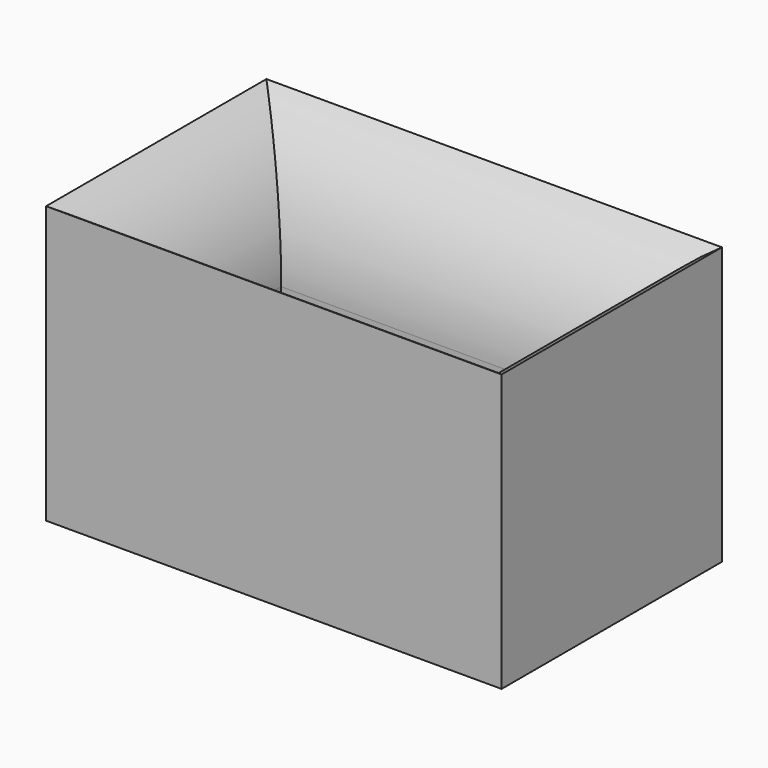
from build123d import *

# Parameters (mm, degrees)
F0_W         = 77.9829304665
F0_H         = 47.1442025155
F1_DEPTH     = 50.8
F2_T         = -12.7
F3_T1_DEPTH  = 52.5829304665
F3_T3_DEPTH  = 21.7442025155
F3_T9_DEPTH  = 116.0829304665
F3_T15_DEPTH = 85.2442025155
F3_T24_DEPTH = 116.0829304665
F3_T30_DEPTH = 85.2442025155
F3_T39_DEPTH = 116.0829304665
F3_T45_DEPTH = 85.2442025155
F3_T54_DEPTH = 85.2442025155
F3_T60_DEPTH = 116.0829304665


# Not quite as in the source:
# - a fillet or chamfer that OpenCascade refuses, or shapes differently, is made with other operations: its cross-section is extruded or revolved along the edge and cut away or added


with BuildPart() as f1:
    # F0 (on Top) → F1 (new body)
    with BuildSketch(Plane.XY):
        with Locations((25.9893098846, -0.1163231209)):
            Rectangle(F0_W, F0_H)
    extrude(amount=F1_DEPTH)

    # F2
    f2_openings = [f1.faces().sort_by_distance(p)[0] for p in [
        (25.98931, -0.116323, 50.8),
    ]]
    offset(amount=F2_T, openings=f2_openings)

    # F3: fillet of radius 25.4 on 4 edges, made by hand

    # F3_s2 → F3_t1 (cut)
    with BuildSketch(Plane.YZ.offset(-0.3021553487)):
        with BuildLine():
            ThreePointArc((36.1557781368, 50.8), (18.1952658947, 43.3605122421), (10.7557781368, 25.4))
            Line((10.7557781368, 25.4), (10.7557781368, 50.8))
            Line((10.7557781368, 50.8), (36.1557781368, 50.8))
        make_face()
        with BuildLine():
            ThreePointArc((-36.3884243786, 50.8), (-18.4279121365, 43.3605122421), (-10.9884243786, 25.4))
            Line((-10.9884243786, 25.4), (-10.9884243786, 50.8))
            Line((-10.9884243786, 50.8), (-36.3884243786, 50.8))
        make_face()
    extrude(amount=F3_T1_DEPTH, mode=Mode.SUBTRACT)

    # F3_s4 → F3_t3 (cut)
    with BuildSketch(Plane.XZ.offset(-10.7557781368)):
        with BuildLine():
            ThreePointArc((-25.7021553487, 50.8), (-7.7416431065, 43.3605122421), (-0.3021553487, 25.4))
            Line((-0.3021553487, 25.4), (-0.3021553487, 50.8))
            Line((-0.3021553487, 50.8), (-25.7021553487, 50.8))
        make_face()
        with BuildLine():
            ThreePointArc((77.6807751179, 50.8), (59.7202628757, 43.3605122421), (52.2807751179, 25.4))
            Line((52.2807751179, 25.4), (52.2807751179, 50.8))
            Line((52.2807751179, 50.8), (77.6807751179, 50.8))
        make_face()
    extrude(amount=F3_T3_DEPTH, mode=Mode.SUBTRACT)


with BuildPart() as f3_tool7:
    # F3_s8 → F3_t9 (new body)
    with BuildSketch(Plane.YZ.offset(115.7807751179)):
        with BuildLine():
            ThreePointArc((36.1557781368, 50.8), (18.1952658947, 43.3605122421), (10.7557781368, 25.4))
            Line((10.7557781368, 25.4), (10.7557781368, 50.8))
            Line((10.7557781368, 50.8), (36.1557781368, 50.8))
        make_face()
    extrude(amount=-F3_T9_DEPTH)

    split(bisect_by=Plane.XZ.offset(-23.4557781368), keep=Keep.TOP)

    split(bisect_by=Plane.YZ.offset(64.9807751179), keep=Keep.BOTTOM)

    split(bisect_by=Plane.YZ.offset(52.2807751179), keep=Keep.TOP)


with BuildPart() as f3_tool13:
    # F3_s14 → F3_t15 (new body)
    with BuildSketch(Plane.XZ.offset(10.9884243786)):
        with BuildLine():
            ThreePointArc((77.6807751179, 50.8), (59.7202628757, 43.3605122421), (52.2807751179, 25.4))
            Line((52.2807751179, 25.4), (52.2807751179, 50.8))
            Line((52.2807751179, 50.8), (77.6807751179, 50.8))
        make_face()
    extrude(amount=-F3_T15_DEPTH)

    split(bisect_by=Plane.XZ.offset(-23.4557781368), keep=Keep.TOP)

    split(bisect_by=Plane.YZ.offset(64.9807751179), keep=Keep.BOTTOM)

    split(bisect_by=Plane.XZ.offset(-10.7557781368), keep=Keep.BOTTOM)


with BuildPart() as f3_tool7_1:
    add(f3_tool7.part)

    # F3_t19: intersect F3_tool13
    add(f3_tool13.part, mode=Mode.INTERSECT)


with BuildPart() as f1_1:
    add(f1.part)

    # F3_t5: cut F3_tool7
    add(f3_tool7_1.part, mode=Mode.SUBTRACT)


with BuildPart() as f3_tool22:
    # F3_s23 → F3_t24 (new body)
    with BuildSketch(Plane.YZ.offset(52.2807751179)):
        with BuildLine():
            ThreePointArc((36.1557781368, 50.8), (18.1952658947, 43.3605122421), (10.7557781368, 25.4))
            Line((10.7557781368, 25.4), (10.7557781368, 50.8))
            Line((10.7557781368, 50.8), (36.1557781368, 50.8))
        make_face()
    extrude(amount=-F3_T24_DEPTH)

    split(bisect_by=Plane.XZ.offset(-23.4557781368), keep=Keep.TOP)

    split(bisect_by=Plane.YZ.offset(-13.0021553487), keep=Keep.TOP)

    split(bisect_by=Plane.YZ.offset(-0.3021553487), keep=Keep.BOTTOM)


with BuildPart() as f3_tool28:
    # F3_s29 → F3_t30 (new body)
    with BuildSketch(Plane.XZ.offset(-74.2557781368)):
        with BuildLine():
            ThreePointArc((-25.7021553487, 50.8), (-7.7416431065, 43.3605122421), (-0.3021553487, 25.4))
            Line((-0.3021553487, 25.4), (-0.3021553487, 50.8))
            Line((-0.3021553487, 50.8), (-25.7021553487, 50.8))
        make_face()
    extrude(amount=F3_T30_DEPTH)

    split(bisect_by=Plane.XZ.offset(-23.4557781368), keep=Keep.TOP)

    split(bisect_by=Plane.YZ.offset(-13.0021553487), keep=Keep.TOP)

    split(bisect_by=Plane.XZ.offset(-10.7557781368), keep=Keep.BOTTOM)


with BuildPart() as f3_tool22_1:
    add(f3_tool22.part)

    # F3_t34: intersect F3_tool28
    add(f3_tool28.part, mode=Mode.INTERSECT)


with BuildPart() as f1_2:
    add(f1_1.part)

    # F3_t20: cut F3_tool22
    add(f3_tool22_1.part, mode=Mode.SUBTRACT)


with BuildPart() as f3_tool37:
    # F3_s38 → F3_t39 (new body)
    with BuildSketch(Plane.YZ.offset(-63.8021553487)):
        with BuildLine():
            ThreePointArc((-36.3884243786, 50.8), (-18.4279121365, 43.3605122421), (-10.9884243786, 25.4))
            Line((-10.9884243786, 25.4), (-10.9884243786, 50.8))
            Line((-10.9884243786, 50.8), (-36.3884243786, 50.8))
        make_face()
    extrude(amount=F3_T39_DEPTH)

    split(bisect_by=Plane.YZ.offset(-13.0021553487), keep=Keep.TOP)

    split(bisect_by=Plane.XZ.offset(23.6884243786), keep=Keep.BOTTOM)

    split(bisect_by=Plane.YZ.offset(-0.3021553487), keep=Keep.BOTTOM)


with BuildPart() as f3_tool43:
    # F3_s44 → F3_t45 (new body)
    with BuildSketch(Plane.XZ.offset(-10.7557781368)):
        with BuildLine():
            ThreePointArc((-25.7021553487, 50.8), (-7.7416431065, 43.3605122421), (-0.3021553487, 25.4))
            Line((-0.3021553487, 25.4), (-0.3021553487, 50.8))
            Line((-0.3021553487, 50.8), (-25.7021553487, 50.8))
        make_face()
    extrude(amount=F3_T45_DEPTH)

    split(bisect_by=Plane.YZ.offset(-13.0021553487), keep=Keep.TOP)

    split(bisect_by=Plane.XZ.offset(23.6884243786), keep=Keep.BOTTOM)

    split(bisect_by=Plane.XZ.offset(10.9884243786), keep=Keep.TOP)


with BuildPart() as f3_tool37_1:
    add(f3_tool37.part)

    # F3_t49: intersect F3_tool43
    add(f3_tool43.part, mode=Mode.INTERSECT)


with BuildPart() as f1_3:
    add(f1_2.part)

    # F3_t35: cut F3_tool37
    add(f3_tool37_1.part, mode=Mode.SUBTRACT)


with BuildPart() as f3_tool52:
    # F3_s53 → F3_t54 (new body)
    with BuildSketch(Plane.XZ.offset(74.4884243786)):
        with BuildLine():
            ThreePointArc((77.6807751179, 50.8), (59.7202628757, 43.3605122421), (52.2807751179, 25.4))
            Line((52.2807751179, 25.4), (52.2807751179, 50.8))
            Line((52.2807751179, 50.8), (77.6807751179, 50.8))
        make_face()
    extrude(amount=-F3_T54_DEPTH)

    split(bisect_by=Plane.XZ.offset(23.6884243786), keep=Keep.BOTTOM)

    split(bisect_by=Plane.YZ.offset(64.9807751179), keep=Keep.BOTTOM)

    split(bisect_by=Plane.XZ.offset(10.9884243786), keep=Keep.TOP)


with BuildPart() as f3_tool58:
    # F3_s59 → F3_t60 (new body)
    with BuildSketch(Plane.YZ.offset(-0.3021553487)):
        with BuildLine():
            ThreePointArc((-36.3884243786, 50.8), (-18.4279121365, 43.3605122421), (-10.9884243786, 25.4))
            Line((-10.9884243786, 25.4), (-10.9884243786, 50.8))
            Line((-10.9884243786, 50.8), (-36.3884243786, 50.8))
        make_face()
    extrude(amount=F3_T60_DEPTH)

    split(bisect_by=Plane.XZ.offset(23.6884243786), keep=Keep.BOTTOM)

    split(bisect_by=Plane.YZ.offset(64.9807751179), keep=Keep.BOTTOM)

    split(bisect_by=Plane.YZ.offset(52.2807751179), keep=Keep.TOP)


with BuildPart() as f3_tool52_1:
    add(f3_tool52.part)

    # F3_t64: intersect F3_tool58
    add(f3_tool58.part, mode=Mode.INTERSECT)


with BuildPart() as f1_4:
    add(f1_3.part)

    # F3_t50: cut F3_tool52
    add(f3_tool52_1.part, mode=Mode.SUBTRACT)


solid = f1_4.part
